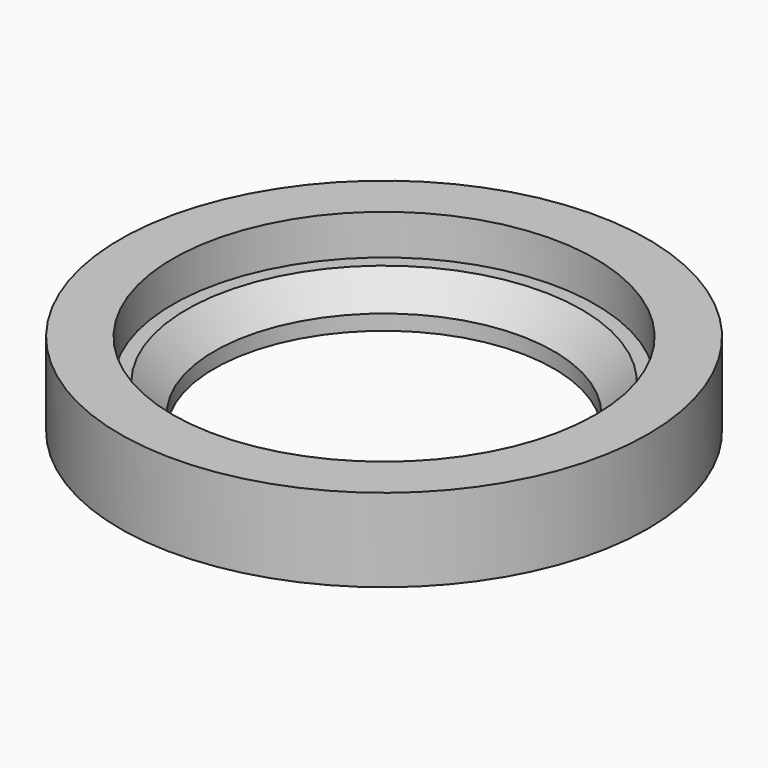
from build123d import *

# Parameters (mm, degrees)
F0_R     = 19.05
F1_DEPTH = 6
F2_R     = 12.25
F3_DEPTH = 6
F4_R     = 15.25
F5_DEPTH = 2.9
F6_SIZE  = 2


# Not quite as in the source:
# - a feature names something its author has since deleted; it is built from what else it names


with BuildPart() as f1:
    # F0 (on Top) → F1 (new body)
    with BuildSketch(Plane.XY):
        Circle(F0_R)
    extrude(amount=F1_DEPTH)

    # F2 (on face) → F3 (cut)
    with BuildSketch(Plane.XY.offset(6)):
        Circle(F2_R)
    extrude(amount=-F3_DEPTH, mode=Mode.SUBTRACT)

    # F4 (on face) → F5 (cut)
    with BuildSketch(Plane.XY.offset(6)):
        Circle(F4_R)
    extrude(amount=-F5_DEPTH, mode=Mode.SUBTRACT)

    # F6
    f6_edges = [f1.edges().sort_by_distance(p)[0] for p in [
        (-12.25, 0, 3.1),
    ]]
    chamfer(f6_edges, length=F6_SIZE)


solid = f1.part
